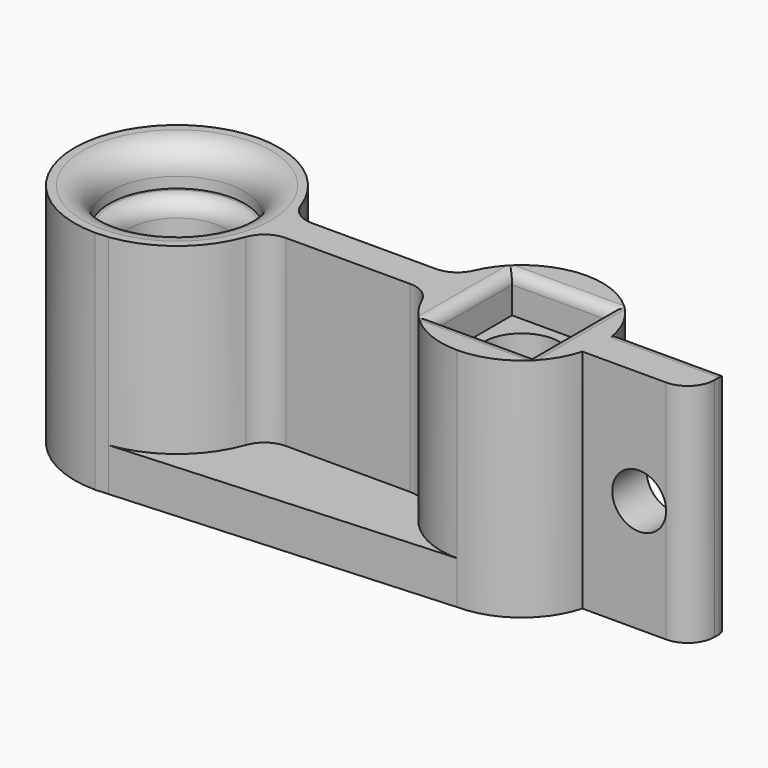
from build123d import *

# Parameters (mm, degrees)
F1_DEPTH       = 21
F1_DEPTH_BACK  = 21
F3_DEPTH       = 34
F4_R           = 6
F4_R_2         = 7
F5_DEPTH       = 42
F6_R           = 9
F6_R_2         = 6
F7_DEPTH       = 22
F8_W           = 18
F8_H           = 18
F8_R           = 7
F9_DEPTH       = 7
F10_R          = 12.5
F11_DEPTH      = 7
F12_R          = 5
F13_DEPTH      = 8
F13_DEPTH_BACK = 8
F14_R          = 4.99999
F15_T1_DEPTH   = 18
F15_T3_DEPTH   = 18
F15_T5_DEPTH   = 52
F15_T10_DEPTH  = 30.5431677052
F15_S11_R      = 15
F15_T12_DEPTH  = 17
F15_T17_DEPTH  = 23
F15_T21_DEPTH  = 23
F15_T28_DEPTH  = 23
F15_T32_DEPTH  = 23
F15_T39_DEPTH  = 23
F15_T43_DEPTH  = 23
F15_T50_DEPTH  = 23
F15_T54_DEPTH  = 23
F16_R          = 2.99999


# Not quite as in the source:
# - a fillet or chamfer that OpenCascade refuses, or shapes differently, is made with other operations: its cross-section is extruded or revolved along the edge and cut away or added
# - a fillet or chamfer is up to 0.001 mm smaller than in the source, because OpenCascade refuses the exact size


with BuildPart() as f1:
    # F0 (on Top) → F1 (new body, two sides)
    with BuildSketch(Plane.XY) as f1_sk:
        with BuildLine():
            Line((4.0776433051, 15), (-57.5565979401, 18.8521400778))
            Line((-57.5565979401, 18.8521400778), (-59.9223566949, 19))
            ThreePointArc((-59.9223566949, 19), (-78.9223566949, 0), (-59.9223566949, -19))
            Line((-59.9223566949, -19), (-57.5565979401, -18.8521400778))
            Line((-57.5565979401, -18.8521400778), (4.0776433051, -15))
            ThreePointArc((4.0776433051, -15), (13.1605943674, -11.9373363863), (18.5344755999, -4))
            ThreePointArc((18.5344755999, -4), (19.0776433051, 0), (18.5344755999, 4))
            ThreePointArc((18.5344755999, 4), (13.1605943674, 11.9373363863), (4.0776433051, 15))
        make_face()
        with BuildLine():
            Line((39.0776433051, 4), (18.5344755999, 4))
            ThreePointArc((18.5344755999, 4), (19.0776433051, 0), (18.5344755999, -4))
            Line((18.5344755999, -4), (39.0776433051, -4))
            Line((39.0776433051, -4), (39.0776433051, 4))
        make_face()
    extrude(amount=F1_DEPTH)
    extrude(f1_sk.sketch, amount=-F1_DEPTH_BACK)

    # F2 (on face) → F3 (cut)
    with BuildSketch(Plane.XY.offset(21)):
        with BuildLine():
            Line((-57.5565979401, -18.8521400778), (-59.9223566949, -19))
            ThreePointArc((-59.9223566949, -19), (-58.737169258, -18.9629989912), (-57.5565979401, -18.8521400778))
        make_face()
        with BuildLine():
            ThreePointArc((-41.1606936556, -3), (-46.7157456922, -13.6596275872), (-57.5565979401, -18.8521400778))
            Line((-57.5565979401, -18.8521400778), (4.0776433051, -15))
            ThreePointArc((4.0776433051, -15), (-5.4091896754, -11.6189500386), (-10.6192951516, -3))
            Line((-10.6192951516, -3), (-41.1606936556, -3))
        make_face()
        with BuildLine():
            Line((-59.9223566949, 19), (-57.5565979401, 18.8521400778))
            ThreePointArc((-57.5565979401, 18.8521400778), (-58.737169258, 18.9629989912), (-59.9223566949, 19))
        make_face()
        with BuildLine():
            ThreePointArc((-10.6192951516, 3), (-5.4091896754, 11.6189500386), (4.0776433051, 15))
            Line((4.0776433051, 15), (-57.5565979401, 18.8521400778))
            ThreePointArc((-57.5565979401, 18.8521400778), (-46.7157456922, 13.6596275872), (-41.1606936556, 3))
            Line((-41.1606936556, 3), (-10.6192951516, 3))
        make_face()
    extrude(amount=-F3_DEPTH, mode=Mode.SUBTRACT)

    # F4 (on face) → F5 (cut)
    with BuildSketch(Plane.XY.offset(21)):
        with Locations((-59.9223566949, 0)):
            Circle(F4_R)
        with Locations((4.0776433051, 0)):
            Circle(F4_R_2)
    extrude(amount=-F5_DEPTH, mode=Mode.SUBTRACT)

    # F6 (on face) → F7 (cut)
    with BuildSketch(Plane.XY.offset(21)):
        with Locations((-59.9223566949, 0)):
            Circle(F6_R)
        with Locations((-59.9223566949, 0)):
            Circle(F6_R_2, mode=Mode.SUBTRACT)
    extrude(amount=-F7_DEPTH, mode=Mode.SUBTRACT)

    # F8 (on face) → F9 (cut)
    with BuildSketch(Plane.XY.offset(21)):
        with Locations((4.0776433051, 0)):
            Rectangle(F8_W, F8_H)
        with Locations((4.0776433051, 0)):
            Circle(F8_R, mode=Mode.SUBTRACT)
    extrude(amount=-F9_DEPTH, mode=Mode.SUBTRACT)

    # F10 (on face) → F11 (cut)
    with BuildSketch(Plane.XY.offset(21)):
        with Locations((-59.9223566949, 0)):
            Circle(F10_R)
    extrude(amount=-F11_DEPTH, mode=Mode.SUBTRACT)

    # F12 (on face) → F13 (cut, two sides)
    with BuildSketch(Plane.XZ.offset(4)) as f13_sk:
        with Locations((29.0776433051, 0)):
            Circle(F12_R)
    extrude(amount=-F13_DEPTH, mode=Mode.SUBTRACT)
    extrude(f13_sk.sketch, amount=F13_DEPTH_BACK, mode=Mode.SUBTRACT)

    # F14 (radius 5 in the source; OpenCascade refuses exactly that, so slightly less here)
    f14_edges = [f1.edges().sort_by_distance(p)[0] for p in [
        (-41.160694, -3, 4),
        (-10.619295, -3, 4),
        (-10.619295, 3, 4),
        (-41.160694, 3, 4),
        (-72.422357, 0, 21),
        (39.077643, -4, 0),
    ]]
    fillet(f14_edges, radius=F14_R)

    # F15: fillet of radius 2 on 6 edges, made by hand

    # F15_s2 → F15_t1 (cut)
    with BuildSketch(Plane.XZ.offset(-9)):
        with BuildLine():
            ThreePointArc((-6.9223566949, 21), (-5.5081431326, 20.4142135624), (-4.9223566949, 19))
            Line((-4.9223566949, 19), (-4.9223566949, 21))
            Line((-4.9223566949, 21), (-6.9223566949, 21))
        make_face()
        with BuildLine():
            ThreePointArc((15.0776433051, 21), (13.6634297427, 20.4142135624), (13.0776433051, 19))
            Line((13.0776433051, 19), (13.0776433051, 21))
            Line((13.0776433051, 21), (15.0776433051, 21))
        make_face()
    extrude(amount=F15_T1_DEPTH, mode=Mode.SUBTRACT)

    # F15_s4 → F15_t3 (cut)
    with BuildSketch(Plane.YZ.offset(-4.9223566949)):
        with BuildLine():
            ThreePointArc((11, 21), (9.5857864376, 20.4142135624), (9, 19))
            Line((9, 19), (9, 21))
            Line((9, 21), (11, 21))
        make_face()
        with BuildLine():
            ThreePointArc((-11, 21), (-9.5857864376, 20.4142135624), (-9, 19))
            Line((-9, 19), (-9, 21))
            Line((-9, 21), (-11, 21))
        make_face()
    extrude(amount=F15_T3_DEPTH, mode=Mode.SUBTRACT)

    # F15_s6 → F15_t5 (cut)
    with BuildSketch(Plane.XY.offset(-26)):
        with BuildLine():
            ThreePointArc((37.0776433051, 4), (38.4918568674, 3.4142135624), (39.0776433051, 2))
            Line((39.0776433051, 2), (39.0776433051, 4))
            Line((39.0776433051, 4), (37.0776433051, 4))
        make_face()
    extrude(amount=F15_T5_DEPTH, mode=Mode.SUBTRACT)


with BuildPart() as f15_tool8:
    # F15_s9 → F15_t10 (new body)
    with BuildSketch(Plane.YZ.offset(44.0776433051)):
        with BuildLine():
            ThreePointArc((2, 21), (3.4142135624, 20.4142135624), (4, 19))
            Line((4, 19), (4, 21))
            Line((4, 21), (2, 21))
        make_face()
    extrude(amount=-F15_T10_DEPTH)

    # F15_s11 → F15_t12 (cut, symmetric)
    with BuildSketch(Plane.XY.offset(20)):
        with Locations((4.0776433051, 0)):
            Circle(F15_S11_R)
    extrude(amount=F15_T12_DEPTH, both=True, mode=Mode.SUBTRACT)


with BuildPart() as f1_1:
    add(f1.part)

    # F15_t7: cut F15_tool8
    add(f15_tool8.part, mode=Mode.SUBTRACT)


with BuildPart() as f15_tool15:
    # F15_s16 → F15_t17 (new body)
    with BuildSketch(Plane.XZ.offset(-14)):
        with BuildLine():
            ThreePointArc((-6.9223566949, 21), (-5.5081431326, 20.4142135624), (-4.9223566949, 19))
            Line((-4.9223566949, 19), (-4.9223566949, 21))
            Line((-4.9223566949, 21), (-6.9223566949, 21))
        make_face()
    extrude(amount=F15_T17_DEPTH)

    split(bisect_by=Plane.XZ.offset(-9), keep=Keep.BOTTOM)


with BuildPart() as f15_tool19:
    # F15_s20 → F15_t21 (new body)
    with BuildSketch(Plane.YZ.offset(13.0776433051)):
        with BuildLine():
            ThreePointArc((11, 21), (9.5857864376, 20.4142135624), (9, 19))
            Line((9, 19), (9, 21))
            Line((9, 21), (11, 21))
        make_face()
    extrude(amount=-F15_T21_DEPTH)

    split(bisect_by=Plane.YZ.offset(-4.9223566949), keep=Keep.BOTTOM)


with BuildPart() as f15_tool15_1:
    add(f15_tool15.part)

    # F15_t23: intersect F15_tool19
    add(f15_tool19.part, mode=Mode.INTERSECT)


with BuildPart() as f1_2:
    add(f1_1.part)

    # F15_t13: cut F15_tool15
    add(f15_tool15_1.part, mode=Mode.SUBTRACT)


with BuildPart() as f15_tool26:
    # F15_s27 → F15_t28 (new body)
    with BuildSketch(Plane.YZ.offset(-9.9223566949)):
        with BuildLine():
            ThreePointArc((-11, 21), (-9.5857864376, 20.4142135624), (-9, 19))
            Line((-9, 19), (-9, 21))
            Line((-9, 21), (-11, 21))
        make_face()
    extrude(amount=F15_T28_DEPTH)

    split(bisect_by=Plane.YZ.offset(-4.9223566949), keep=Keep.BOTTOM)


with BuildPart() as f15_tool30:
    # F15_s31 → F15_t32 (new body)
    with BuildSketch(Plane.XZ.offset(-9)):
        with BuildLine():
            ThreePointArc((-6.9223566949, 21), (-5.5081431326, 20.4142135624), (-4.9223566949, 19))
            Line((-4.9223566949, 19), (-4.9223566949, 21))
            Line((-4.9223566949, 21), (-6.9223566949, 21))
        make_face()
    extrude(amount=F15_T32_DEPTH)

    split(bisect_by=Plane.XZ.offset(9), keep=Keep.TOP)


with BuildPart() as f15_tool26_1:
    add(f15_tool26.part)

    # F15_t34: intersect F15_tool30
    add(f15_tool30.part, mode=Mode.INTERSECT)


with BuildPart() as f1_3:
    add(f1_2.part)

    # F15_t24: cut F15_tool26
    add(f15_tool26_1.part, mode=Mode.SUBTRACT)


with BuildPart() as f15_tool37:
    # F15_s38 → F15_t39 (new body)
    with BuildSketch(Plane.XZ.offset(9)):
        with BuildLine():
            ThreePointArc((15.0776433051, 21), (13.6634297427, 20.4142135624), (13.0776433051, 19))
            Line((13.0776433051, 19), (13.0776433051, 21))
            Line((13.0776433051, 21), (15.0776433051, 21))
        make_face()
    extrude(amount=-F15_T39_DEPTH)

    split(bisect_by=Plane.XZ.offset(-9), keep=Keep.BOTTOM)


with BuildPart() as f15_tool41:
    # F15_s42 → F15_t43 (new body)
    with BuildSketch(Plane.YZ.offset(18.0776433051)):
        with BuildLine():
            ThreePointArc((11, 21), (9.5857864376, 20.4142135624), (9, 19))
            Line((9, 19), (9, 21))
            Line((9, 21), (11, 21))
        make_face()
    extrude(amount=-F15_T43_DEPTH)

    split(bisect_by=Plane.YZ.offset(13.0776433051), keep=Keep.TOP)


with BuildPart() as f15_tool37_1:
    add(f15_tool37.part)

    # F15_t45: intersect F15_tool41
    add(f15_tool41.part, mode=Mode.INTERSECT)


with BuildPart() as f1_4:
    add(f1_3.part)

    # F15_t35: cut F15_tool37
    add(f15_tool37_1.part, mode=Mode.SUBTRACT)


with BuildPart() as f15_tool48:
    # F15_s49 → F15_t50 (new body)
    with BuildSketch(Plane.YZ.offset(-4.9223566949)):
        with BuildLine():
            ThreePointArc((-11, 21), (-9.5857864376, 20.4142135624), (-9, 19))
            Line((-9, 19), (-9, 21))
            Line((-9, 21), (-11, 21))
        make_face()
    extrude(amount=F15_T50_DEPTH)

    split(bisect_by=Plane.YZ.offset(13.0776433051), keep=Keep.TOP)


with BuildPart() as f15_tool52:
    # F15_s53 → F15_t54 (new body)
    with BuildSketch(Plane.XZ.offset(14)):
        with BuildLine():
            ThreePointArc((15.0776433051, 21), (13.6634297427, 20.4142135624), (13.0776433051, 19))
            Line((13.0776433051, 19), (13.0776433051, 21))
            Line((13.0776433051, 21), (15.0776433051, 21))
        make_face()
    extrude(amount=-F15_T54_DEPTH)

    split(bisect_by=Plane.XZ.offset(9), keep=Keep.TOP)


with BuildPart() as f15_tool48_1:
    add(f15_tool48.part)

    # F15_t56: intersect F15_tool52
    add(f15_tool52.part, mode=Mode.INTERSECT)


with BuildPart() as f1_5:
    add(f1_4.part)

    # F15_t46: cut F15_tool48
    add(f15_tool48_1.part, mode=Mode.SUBTRACT)

    # F16 (radius 3 in the source; OpenCascade refuses exactly that, so slightly less here)
    f16_edges = [f1_5.edges().sort_by_distance(p)[0] for p in [
        (-68.922357, 0, 14),
        (-65.922357, 0, -1),
    ]]
    fillet(f16_edges, radius=F16_R)


solid = f1_5.part
